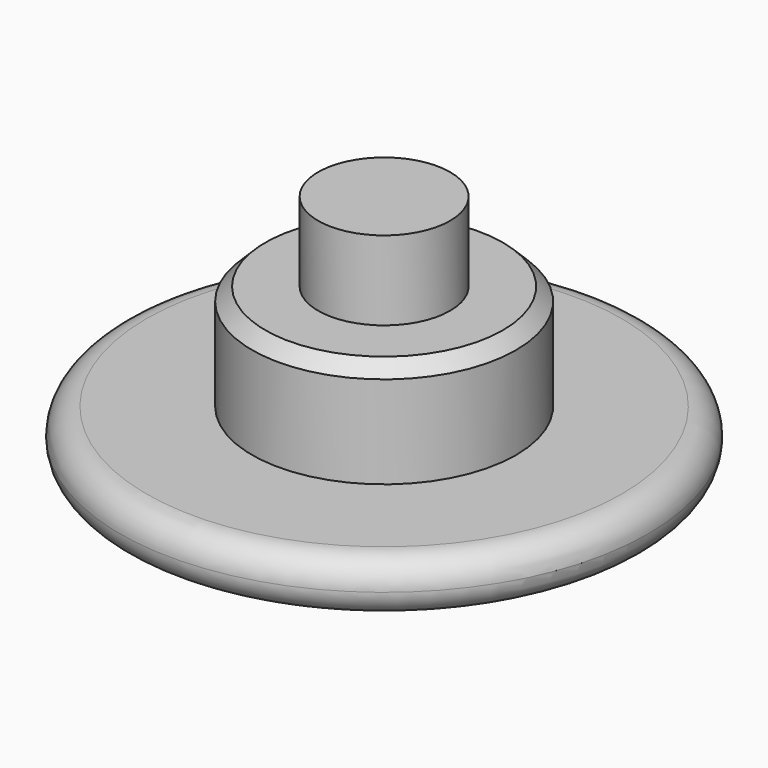
from build123d import *

# Parameters (mm, degrees)
F0_R     = 10
F1_DEPTH = 2
F2_R     = 5
F3_DEPTH = 4
F4_SIZE  = 0.5
F5_R     = 0.99999
F6_R     = 2.5
F7_DEPTH = 3


# Not quite as in the source:
# - a fillet or chamfer is up to 0.001 mm smaller than in the source, because OpenCascade refuses the exact size


with BuildPart() as f1:
    # F0 (on Top) → F1 (new body)
    with BuildSketch(Plane.XY):
        Circle(F0_R)
    extrude(amount=F1_DEPTH)

    # F2 (on face) → F3 (join)
    with BuildSketch(Plane.XY.offset(2)):
        Circle(F2_R)
    extrude(amount=F3_DEPTH)

    # F4
    f4_edges = [f1.edges().sort_by_distance(p)[0] for p in [
        (-5, 0, 6),
    ]]
    chamfer(f4_edges, length=F4_SIZE)

    # F5 (radius 1 in the source; OpenCascade refuses exactly that, so slightly less here)
    f5_edges = [f1.edges().sort_by_distance(p)[0] for p in [
        (-10, 0, 0),
        (-10, 0, 2),
    ]]
    fillet(f5_edges, radius=F5_R)

    # F6 (on face) → F7 (join)
    with BuildSketch(Plane.XY.offset(6)):
        Circle(F6_R)
    extrude(amount=F7_DEPTH)


solid = f1.part
